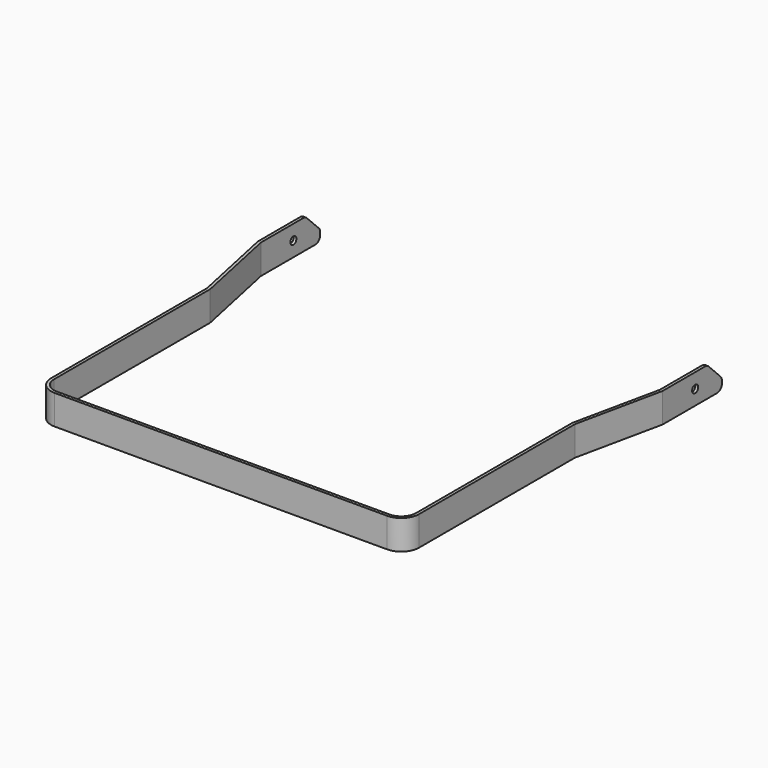
from build123d import *

# Parameters (mm, degrees)
F1_DEPTH = 25.4
F3_D     = 6.5278
F4_SIZE2 = 15.875
F4_SIZE  = 15.875
F5_R     = 5.08


with BuildPart() as f1:
    # F0 (on Top) → F1 (new body)
    with BuildSketch(Plane.XY):
        with BuildLine():
            Line((-65.826073072, 23.3069159811), (-65.826073072, 86.8069159811))
            Line((-65.826073072, 86.8069159811), (-68.366073072, 86.8069159811))
            Line((-68.366073072, 86.8069159811), (-68.366073072, 23.0399512236))
            Line((-68.366073072, 23.0399512236), (-52.5691465571, -51.2787448955))
            Line((-52.5691465571, -51.2787448955), (-52.5691465571, -218.829580138))
            ThreePointArc((-52.5691465571, -218.829580138), (-48.1054539024, -229.6058874832), (-37.3291465571, -234.069580138))
            Line((-37.3291465571, -234.069580138), (248.4208534429, -234.069580138))
            ThreePointArc((248.4208534429, -234.069580138), (259.1971607882, -229.6058874832), (263.6608534429, -218.829580138))
            Line((263.6608534429, -218.829580138), (263.6608534429, -51.2787448955))
            Line((263.6608534429, -51.2787448955), (279.4577799578, 23.0399512236))
            Line((279.4577799578, 23.0399512236), (279.4577799578, 86.8069159811))
            Line((279.4577799578, 86.8069159811), (276.9177799578, 86.8069159811))
            Line((276.9177799578, 86.8069159811), (276.9177799578, 23.3069159811))
            Line((276.9177799578, 23.3069159811), (261.1208534429, -51.011780138))
            Line((261.1208534429, -51.011780138), (261.1208534429, -218.829580138))
            ThreePointArc((261.1208534429, -218.829580138), (257.401109564, -227.809836259), (248.4208534429, -231.529580138))
            Line((248.4208534429, -231.529580138), (-37.3291465571, -231.529580138))
            ThreePointArc((-37.3291465571, -231.529580138), (-46.3094026781, -227.809836259), (-50.0291465571, -218.829580138))
            Line((-50.0291465571, -218.829580138), (-50.0291465571, -51.011780138))
            Line((-50.0291465571, -51.011780138), (-65.826073072, 23.3069159811))
        make_face()
    extrude(amount=F1_DEPTH)

    # F3 (through all)
    with Locations(Plane.YZ.offset(279.4577799578)):
        with Locations((58.0538512236, 12.7)):
            Hole(F3_D / 2)

    # F4
    f4_edges = [f1.edges().sort_by_distance(p)[0] for p in [
        (278.18778, 86.806916, 25.4),
        (-67.096073, 86.806916, 25.4),
    ]]
    chamfer(f4_edges, length=F4_SIZE, length2=F4_SIZE2)

    # F5
    f5_edges = [f1.edges().sort_by_distance(p)[0] for p in [
        (-67.096073, 70.931916, 25.4),
        (278.18778, 70.931916, 25.4),
        (278.18778, 86.806916, 9.525),
        (-67.096073, 86.806916, 9.525),
        (-67.096073, 86.806916, 0),
        (278.18778, 86.806916, 0),
    ]]
    fillet(f5_edges, radius=F5_R)


solid = f1.part
